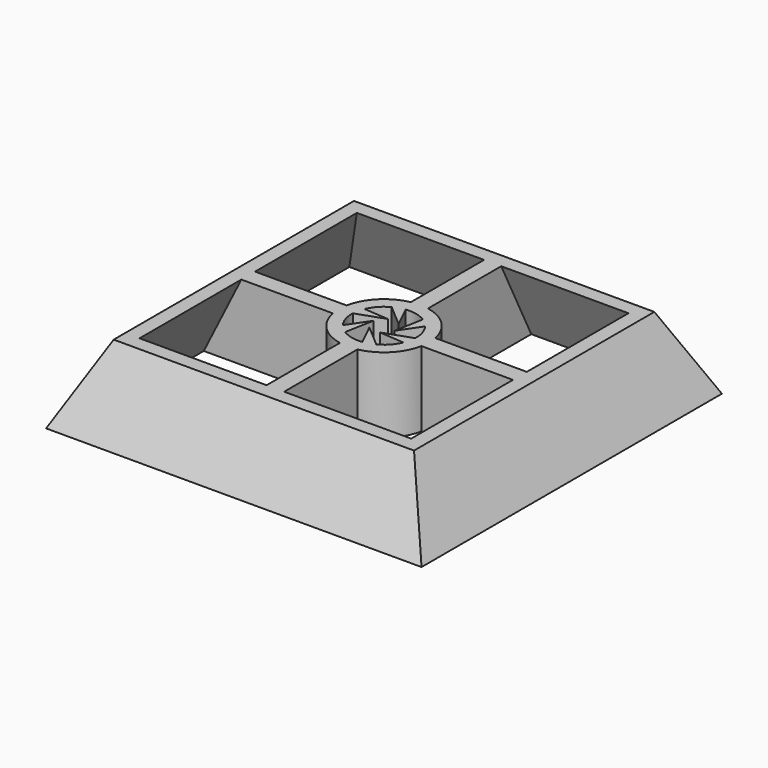
from build123d import *

# Parameters (mm, degrees)
F0_W       = 35
F0_H       = 35
F2_W       = 28
F2_H       = 28
F4_T       = -1.2
F5_R       = 3
F6_DEPTH   = 7
F7_SIZE2   = 3
F7_SIZE    = 6
F7_2_SIZE2 = 3
F7_2_SIZE  = 6
F7_3_SIZE2 = 3
F7_3_SIZE  = 6
F7_4_SIZE2 = 3
F7_4_SIZE  = 6
F10_DEPTH  = 7


# Not quite as in the source:
# - a feature names something its author has since deleted; it is built from what else it names


with BuildPart() as f3:
    # F0 (on Top) → F3 section 0
    with BuildSketch(Plane.XY):
        Rectangle(F0_W, F0_H)
    # F2 (on offset) → F3 section 1
    with BuildSketch(Plane.XY.offset(7)):
        Rectangle(F2_W, F2_H)
    loft()

    # F4
    f4_openings = [f3.faces().sort_by_distance(p)[0] for p in [
        (0, 0, 7),
        (0, 0, 0),
    ]]
    offset(amount=F4_T, openings=f4_openings)


with BuildPart() as f6:
    # F5 (on Top) → F6 (new body, through all)
    with BuildSketch(Plane.XY):
        with BuildLine():
            Line((-16.2, -0.8), (-4.1231056256, -0.8))
            ThreePointArc((-4.1231056256, -0.8), (-2.9768706674, -2.9628096513), (-0.8195121951, -4.1192717514))
            Line((-0.8195121951, -4.1192717514), (-0.8195121951, -16.2))
            Line((-0.8195121951, -16.2), (0.8195121951, -16.2))
            Line((0.8195121951, -16.2), (0.8195121951, -4.1192717514))
            ThreePointArc((0.8195121951, -4.1192717514), (2.9768706674, -2.9628096513), (4.1231056256, -0.8))
            Line((4.1231056256, -0.8), (16.2, -0.8))
            Line((16.2, -0.8), (16.2, 0.8195121951))
            Line((16.2, 0.8195121951), (4.1192717514, 0.8195121951))
            ThreePointArc((4.1192717514, 0.8195121951), (2.9628096513, 2.9768706674), (0.8, 4.1231056256))
            Line((0.8, 4.1231056256), (0.8, 16.2))
            Line((0.8, 16.2), (-0.8, 16.2))
            Line((-0.8, 16.2), (-0.8, 4.1231056256))
            ThreePointArc((-0.8, 4.1231056256), (-2.969848481, 2.969848481), (-4.1231056256, 0.8))
            Line((-4.1231056256, 0.8), (-16.2, 0.8))
            Line((-16.2, 0.8), (-16.2, -0.8))
        make_face()
        Circle(F5_R, mode=Mode.SUBTRACT)
    extrude(amount=F6_DEPTH)

    # F7
    f7_edges = [f6.edges().sort_by_distance(p)[0] for p in [
        (-16.2, 0, 7),
    ]]
    f7_side = f6.faces().sort_by_distance((-16.2, 0, 3.5))[0]
    chamfer(f7_edges, length=F7_SIZE, length2=F7_SIZE2, reference=f7_side)

    # F7#2
    f7_2_edges = [f6.edges().sort_by_distance(p)[0] for p in [
        (0, 16.2, 7),
    ]]
    f7_2_side = f6.faces().sort_by_distance((0, 16.2, 3.5))[0]
    chamfer(f7_2_edges, length=F7_2_SIZE, length2=F7_2_SIZE2, reference=f7_2_side)

    # F7#3
    f7_3_edges = [f6.edges().sort_by_distance(p)[0] for p in [
        (16.2, 0.009756, 7),
    ]]
    f7_3_side = f6.faces().sort_by_distance((16.2, 0.009756, 3.5))[0]
    chamfer(f7_3_edges, length=F7_3_SIZE, length2=F7_3_SIZE2, reference=f7_3_side)

    # F7#4
    f7_4_edges = [f6.edges().sort_by_distance(p)[0] for p in [
        (0, -16.2, 7),
    ]]
    f7_4_side = f6.faces().sort_by_distance((0, -16.2, 3.5))[0]
    chamfer(f7_4_edges, length=F7_4_SIZE, length2=F7_4_SIZE2, reference=f7_4_side)


with BuildPart() as f3_1:
    add(f3.part)

    # F8: union F6
    add(f6.part)

    # F9 (on face) → F10 (join, through all)
    with BuildSketch(Plane.XY.offset(7)):
        with BuildLine():
            Line((0.6612347815, 0.8790725588), (-0.3595485903, 2.9783762038))
            ThreePointArc((-0.3595485903, 2.9783762038), (-0.8973940811, 2.8626358244), (-1.4050598491, 2.6506238549))
            Line((-1.4050598491, 2.6506238549), (0.6612347815, 0.8790725588))
        make_face()
        with BuildLine():
            Line((-0.430681777, 1.0121823981), (-2.7591237497, 1.1778098887))
            ThreePointArc((-2.7591237497, 1.1778098887), (-2.9278123863, 0.6541518408), (-2.9980375188, 0.1084944043))
            Line((-2.9980375188, 0.1084944043), (-0.430681777, 1.0121823981))
        make_face()
        with BuildLine():
            Line((-1.0919165585, 0.1331098393), (-2.3995751593, -1.800566315))
            ThreePointArc((-2.3995751593, -1.800566315), (-2.0304183052, -2.2084839836), (-1.5929776697, -2.5421294507))
            Line((-1.5929776697, -2.5421294507), (-1.0919165585, 0.1331098393))
        make_face()
        with BuildLine():
            Line((-0.6612347815, -0.8790725588), (0.3595485903, -2.9783762038))
            ThreePointArc((0.3595485903, -2.9783762038), (0.8973940811, -2.8626358244), (1.4050598491, -2.6506238549))
            Line((1.4050598491, -2.6506238549), (-0.6612347815, -0.8790725588))
        make_face()
        with BuildLine():
            ThreePointArc((2.7591237497, -1.1778098887), (2.9278123863, -0.6541518408), (2.9980375188, -0.1084944043))
            Line((2.9980375188, -0.1084944043), (0.430681777, -1.0121823981))
            Line((0.430681777, -1.0121823981), (2.7591237497, -1.1778098887))
        make_face()
        with BuildLine():
            ThreePointArc((2.3995751593, 1.800566315), (2.0304183052, 2.2084839836), (1.5929776697, 2.5421294507))
            Line((1.5929776697, 2.5421294507), (1.0919165585, -0.1331098393))
            Line((1.0919165585, -0.1331098393), (2.3995751593, 1.800566315))
        make_face()
    extrude(amount=-F10_DEPTH)


solid = f3_1.part
